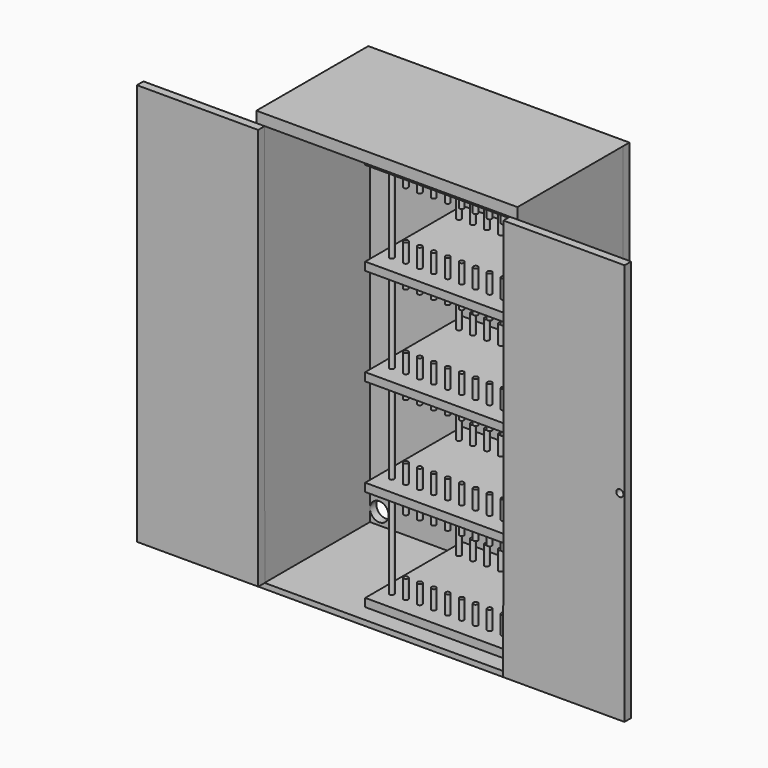
from build123d import *

# Parameters (mm, degrees)
F0_W          = 406.4
F0_H          = 22.225
F1_DEPTH      = 330.2
F3_R          = 6.35
F4_DEPTH      = 563.5752
F4_DEPTH_BACK = 519.1252
F0_W_2        = 330.2
F0_H_2        = 130.175
F0_H_3        = 152.4
F5_DEPTH      = 304.8
F6_W          = 711.1986837864
F6_H          = 1139.7287186623
F6_W_2        = 666.7486837864
F6_H_2        = 1095.2787186623
F7_DEPTH      = 355.6
F7_DEPTH_BACK = 25.4
F9_W          = 711.1986837864
F9_H          = 1139.7287186623
F9_R          = 25.4
F10_DEPTH     = 22.225
F11_DEPTH     = 25.4
F13_R         = 9.525
F14_DEPTH     = 22.225


# Not quite as in the source:
# - a feature names something its author has since deleted; it is built from what else it names


with BuildPart() as f1:
    # F0 (on Front) → F1 (new body)
    with BuildSketch(Plane.XZ):
        with Locations((0, -265.1125)):
            Rectangle(F0_W, F0_H)
    extrude(amount=-F1_DEPTH)

    # F9 (on offset) → F11 (cut)
    with BuildSketch(Plane(origin=(0, 355.6, 0), x_dir=(-1, 0, 0), z_dir=(0, 1, 0))):
        with Locations((431.7003317833, -533.4750243187)):
            Circle(F9_R)
    extrude(amount=-F11_DEPTH, mode=Mode.SUBTRACT)


with BuildPart() as f1b:
    # F0 (on Front) → F1, piece 2 (new body)
    with BuildSketch(Plane.XZ):
        Rectangle(F0_W, F0_H)
    extrude(amount=-F1_DEPTH)

    # F3 (on offset) → F4 (join, two sides)
    with BuildSketch(Plane.XY.offset(11.1125)) as f4_sk:
        with Locations((171.45, 279.4)):
            Circle(F3_R)
        with Locations((171.45, 50.8)):
            Circle(F3_R)
        with Locations((133.35, 279.4)):
            Circle(F3_R)
        with Locations((133.35, 50.8)):
            Circle(F3_R)
        with Locations((95.25, 279.4)):
            Circle(F3_R)
        with Locations((95.25, 50.8)):
            Circle(F3_R)
        with Locations((57.15, 279.4)):
            Circle(F3_R)
        with Locations((57.15, 50.8)):
            Circle(F3_R)
        with Locations((19.05, 279.4)):
            Circle(F3_R)
        with Locations((19.05, 50.8)):
            Circle(F3_R)
        with Locations((-19.05, 279.4)):
            Circle(F3_R)
        with Locations((-19.05, 50.8)):
            Circle(F3_R)
        with Locations((-57.15, 279.4)):
            Circle(F3_R)
        with Locations((-57.15, 50.8)):
            Circle(F3_R)
        with Locations((-95.25, 279.4)):
            Circle(F3_R)
        with Locations((-95.25, 50.8)):
            Circle(F3_R)
        with Locations((-133.35, 279.4)):
            Circle(F3_R)
        with Locations((-133.35, 50.8)):
            Circle(F3_R)
        with Locations((-171.45, 279.4)):
            Circle(F3_R)
        with Locations((-171.45, 50.8)):
            Circle(F3_R)
    extrude(amount=-F4_DEPTH)
    extrude(f4_sk.sketch, amount=F4_DEPTH_BACK)

    # F0 (on Front) → F5 (cut)
    with BuildSketch(Plane.XZ):
        with Locations((0, 392.1125)):
            Rectangle(F0_W_2, F0_H_2)
        with Locations((0, 138.1125)):
            Rectangle(F0_W_2, F0_H_3)
        with Locations((0, -127)):
            Rectangle(F0_W_2, F0_H_3)
        with Locations((0, -403.2377)):
            Rectangle(F0_W_2, F0_H_3)
    extrude(amount=-F5_DEPTH, mode=Mode.SUBTRACT)


with BuildPart() as f1c:
    # F0 (on Front) → F1, piece 3 (new body)
    with BuildSketch(Plane.XZ):
        with Locations((0, 265.1125)):
            Rectangle(F0_W, F0_H)
    extrude(amount=-F1_DEPTH)


with BuildPart() as f1d:
    # F0 (on Front) → F1, piece 4 (new body)
    with BuildSketch(Plane.XZ):
        with Locations((0, 519.1125)):
            Rectangle(F0_W, F0_H)
    extrude(amount=-F1_DEPTH)


with BuildPart() as f1e:
    # F0 (on Front) → F1, piece 5 (new body)
    with BuildSketch(Plane.XZ):
        with Locations((0, -541.3502)):
            Rectangle(F0_W, F0_H)
    extrude(amount=-F1_DEPTH)


with BuildPart() as f7:
    # F6 (on Front) → F7 (new body, two sides)
    with BuildSketch(Plane.XZ) as f7_sk:
        with Locations((-123.7428946018, -11.219650507)):
            Rectangle(F6_W, F6_H)
        with Locations((-123.7428946018, -18.7989179134)):
            Rectangle(F6_W_2, F6_H_2, mode=Mode.SUBTRACT)
    extrude(amount=-F7_DEPTH)
    extrude(f7_sk.sketch, amount=F7_DEPTH_BACK)

    # F9 (on offset) → F10 (join)
    with BuildSketch(Plane(origin=(0, 355.6, 0), x_dir=(-1, 0, 0), z_dir=(0, 1, 0))):
        with Locations((123.7302739382, -11.241105032)):
            Rectangle(F9_W, F9_H)
        with Locations((431.7003317833, -533.4750243187)):
            Circle(F9_R, mode=Mode.SUBTRACT)
    extrude(amount=-F10_DEPTH)

    # F13 (on offset) → F14 (join)
    with BuildSketch(Plane.XZ.offset(25.4)):
        Polygon((-456.5249979496, -566.302716732), (-456.8764567375, 528.7907719612), (-787.0764567375, 528.7907719612), (-786.7249979496, -566.302716732), align=None)
        Polygon((541.3635804176, 528.7907719612), (211.1635804176, 528.7907719612), (210.8121216297, -566.302716732), (541.0121216297, -566.302716732), align=None)
        with Locations((528.51190361, -21.7313145863)):
            Circle(F13_R, mode=Mode.SUBTRACT)
    extrude(amount=F14_DEPTH)


solid = Compound([f1.part, f1b.part, f1c.part, f1d.part, f1e.part, f7.part])
